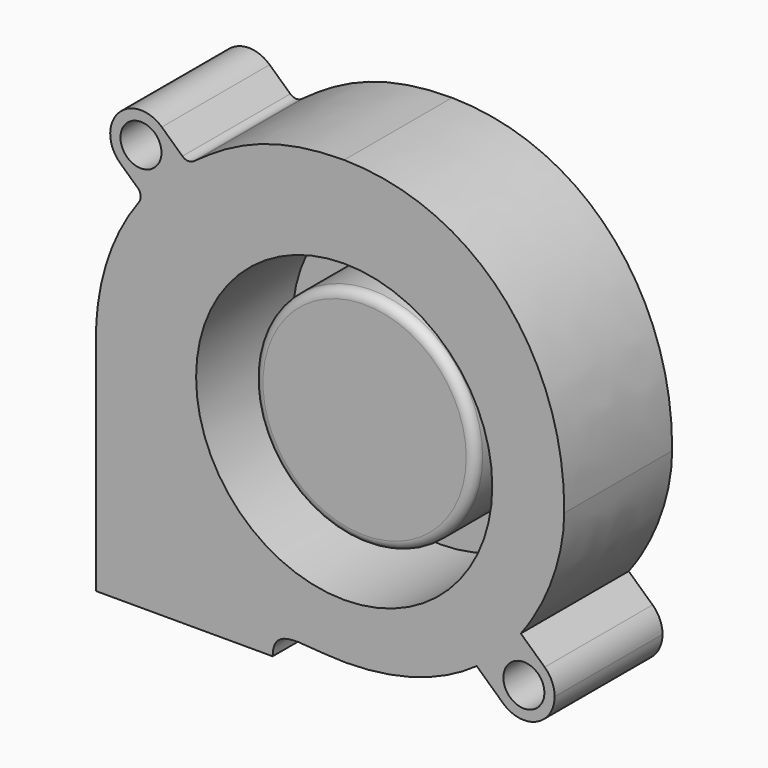
from build123d import *

# Parameters (mm, degrees)
F0_R     = 2.25
F1_DEPTH = 14.8
F0_R_2   = 12.15
F2_DEPTH = 1.6
F3_DEPTH = 12
F4_R     = 1
F5_W     = 17.4
F5_H     = 12.06
F6_DEPTH = 5


with BuildPart() as f1:
    # F0 (on Front) → F1 (new body)
    with BuildSketch(Plane.XZ):
        with BuildLine():
            Line((-27.25, 0), (-27.25, -24.25))
            Line((-27.25, -24.25), (-7.85, -24.25))
            add(Edge.make_bspline(
                [(-7.85, -24.25), (-7.8176427633, -20.8169110119), (-4.3375464156, -22.25), (0, -22.25)],
                knots=[0, 0, 0, 0, 8.1007715682, 8.1007715682, 8.1007715682, 8.1007715682], degree=3))
            add(Edge.make_bspline(
                [(14.5437740109, -17.909216005), (10.9068056005, -20.5097986935), (6.122203429, -22.25), (0, -22.25)],
                knots=[21.4185998801, 21.4185998801, 21.4185998801, 21.4185998801, 32.8372501894, 32.8372501894, 32.8372501894, 32.8372501894], degree=3))
            add(Edge.make_bspline(
                [(19.3821703567, -13.1875596661), (18.0720576154, -14.9154903789), (16.4686462302, -16.5328528348), (14.5437740109, -17.909216005)],
                knots=[15.3752582058, 15.3752582058, 15.3752582058, 15.3752582058, 21.4185998801, 21.4185998801, 21.4185998801, 21.4185998801], degree=3))
            add(Edge.make_bspline(
                [(24.15, 0), (24.15, -3.6795945823), (22.7153133033, -8.7914188713), (19.3821703567, -13.1875596661)],
                knots=[0, 0, 0, 0, 15.3752582058, 15.3752582058, 15.3752582058, 15.3752582058], degree=3))
            add(Edge.make_bspline(
                [(24.15, 0), (24.2929216474, 14.3250608817), (14.8955499753, 26.0717794299), (0, 26.25)],
                knots=[0, 0, 0, 0, 35.6691042781, 35.6691042781, 35.6691042781, 35.6691042781], degree=3))
            add(Edge.make_bspline(
                [(0, 26.25), (-5.135877891, 26.2629323961), (-11.114542158, 24.5071482084), (-16.161044046, 21.0100500089)],
                knots=[0, 0, 0, 0, 16.8847295513, 16.8847295513, 16.8847295513, 16.8847295513], degree=3))
            add(Edge.make_bspline(
                [(-16.161044046, 21.0100500089), (-16.2712231538, 20.9311478534), (-16.3801314978, 20.8526765927), (-16.487850408, 20.7747483814)],
                knots=[16.497992714, 16.497992714, 16.497992714, 16.497992714, 17.0339105302, 17.0339105302, 17.0339105302, 17.0339105302], degree=3))
            add(Edge.make_bspline(
                [(-16.487850408, 20.7747483814), (-16.7124834128, 20.6122397909), (-16.9319438817, 20.4520927797), (-17.1469693705, 20.2953244431)],
                knots=[17.0339105302, 17.0339105302, 17.0339105302, 17.0339105302, 18.1514935909, 18.1514935909, 18.1514935909, 18.1514935909], degree=3))
            add(Edge.make_bspline(
                [(-17.1469693705, 20.2953244431), (-19.1547308604, 18.7732329399), (-20.9874640515, 16.9609662016), (-22.5242380569, 14.8603912213)],
                knots=[17.9984458903, 17.9984458903, 17.9984458903, 17.9984458903, 24.8946681266, 24.8946681266, 24.8946681266, 24.8946681266], degree=3))
            add(Edge.make_bspline(
                [(-22.5242380569, 14.8603912213), (-25.4083045723, 10.9182384112), (-27.25, 5.9606612107), (-27.25, 0)],
                knots=[24.8946681266, 24.8946681266, 24.8946681266, 24.8946681266, 37.836820691, 37.836820691, 37.836820691, 37.836820691], degree=3))
        make_face()
        with BuildLine():
            ThreePointArc((16.25, 0), (-11.4904851943, -11.4904851943), (0, 16.25))
            ThreePointArc((0, 16.25), (11.4904851943, 11.4904851943), (16.25, 0))
        make_face(mode=Mode.SUBTRACT)
        with BuildLine():
            ThreePointArc((-22.6556099396, 16.1880189983), (-22.3361709954, 15.5493145647), (-22.5242380569, 14.8603912213))
            add(Edge.make_bspline(
                [(-17.1469693705, 20.2953244431), (-19.1547308604, 18.7732329399), (-20.9874640515, 16.9609662016), (-22.5242380569, 14.8603912213)],
                knots=[17.9984458903, 17.9984458903, 17.9984458903, 17.9984458903, 24.8946681266, 24.8946681266, 24.8946681266, 24.8946681266], degree=3))
            add(Edge.make_bspline(
                [(-16.5707430692, 20.7208158925), (-16.7643258601, 20.5815997135), (-16.9564357443, 20.4397686985), (-17.1469693705, 20.2953244431)],
                knots=[17.3440044956, 17.3440044956, 17.3440044956, 17.3440044956, 17.9984458903, 17.9984458903, 17.9984458903, 17.9984458903], degree=3))
            ThreePointArc((-16.5707430692, 20.7208158925), (-17.1810656026, 20.5907080667), (-17.7496903525, 20.8477830266))
            Line((-17.7496903525, 20.8477830266), (-20.0190790788, 22.927921795))
            ThreePointArc((-20.0190790788, 22.927921795), (-19.2102914227, 21.7989913577), (-18.924569733, 20.439953271))
            ThreePointArc((-18.924569733, 20.439953271), (-20.9405316464, 17.3506749607), (-24.5800603872, 17.9519847471))
            Line((-24.5800603872, 17.9519847471), (-22.6556099396, 16.1880189983))
        make_face()
        with BuildLine():
            add(Edge.make_bspline(
                [(19.3821703567, -13.1875596661), (18.0720576154, -14.9154903789), (16.4686462302, -16.5328528348), (14.5437740109, -17.909216005)],
                knots=[15.3752582058, 15.3752582058, 15.3752582058, 15.3752582058, 21.4185998801, 21.4185998801, 21.4185998801, 21.4185998801], degree=3))
            Line((14.5437740109, -17.909216005), (17.4389635725, -20.5629685239))
            ThreePointArc((17.4389635725, -20.5629685239), (17.2314857028, -15.7945093458), (21.9999448809, -15.5870314761))
            Line((21.9999448809, -15.5870314761), (19.3821703567, -13.1875596661))
        make_face()
        with BuildLine():
            add(Edge.make_bspline(
                [(-16.5707430692, 20.7208158925), (-16.7643258601, 20.5815997135), (-16.9564357443, 20.4397686985), (-17.1469693705, 20.2953244431)],
                knots=[17.3440044956, 17.3440044956, 17.3440044956, 17.3440044956, 17.9984458903, 17.9984458903, 17.9984458903, 17.9984458903], degree=3))
            add(Edge.make_bspline(
                [(-16.487850408, 20.7747483814), (-16.7124834128, 20.6122397909), (-16.9319438817, 20.4520927797), (-17.1469693705, 20.2953244431)],
                knots=[17.0339105302, 17.0339105302, 17.0339105302, 17.0339105302, 18.1514935909, 18.1514935909, 18.1514935909, 18.1514935909], degree=3))
            ThreePointArc((-16.487850408, 20.7747483814), (-16.5286296346, 20.7467568176), (-16.5707430692, 20.7208158925))
        make_face()
        with BuildLine():
            ThreePointArc((21.9999448809, -15.5870314761), (17.2314857028, -15.7945093458), (17.4389635725, -20.5629685239))
            ThreePointArc((17.4389635725, -20.5629685239), (21.0784923134, -21.1642783104), (23.0944542267, -18.075))
            ThreePointArc((23.0944542267, -18.075), (22.8087325371, -16.7159619133), (21.9999448809, -15.5870314761))
        make_face()
        with Locations((19.7194542267, -18.075)):
            Circle(F0_R, mode=Mode.SUBTRACT)
        with BuildLine():
            ThreePointArc((-20.0190790788, 22.927921795), (-24.787538257, 22.7204439252), (-24.5800603872, 17.9519847471))
            ThreePointArc((-24.5800603872, 17.9519847471), (-20.9405316464, 17.3506749607), (-18.924569733, 20.439953271))
            ThreePointArc((-18.924569733, 20.439953271), (-19.2102914227, 21.7989913577), (-20.0190790788, 22.927921795))
        make_face()
        with Locations((-22.299569733, 20.439953271)):
            Circle(F0_R, mode=Mode.SUBTRACT)
        with BuildLine():
            add(Edge.make_bspline(
                [(0, 26.25), (-8.1731251983, 26.2763401513), (-12.7692289915, 23.4390179358), (-16.161044046, 21.0100500089)],
                knots=[0, 0, 0, 0, 16.497992714, 16.497992714, 16.497992714, 16.497992714], degree=3))
            add(Edge.make_bspline(
                [(0, 26.25), (-5.135877891, 26.2629323961), (-11.114542158, 24.5071482084), (-16.161044046, 21.0100500089)],
                knots=[0, 0, 0, 0, 16.8847295513, 16.8847295513, 16.8847295513, 16.8847295513], degree=3))
        make_face()
    extrude(amount=F1_DEPTH)

    # F0 (on Front) → F2 (join)
    with BuildSketch(Plane.XZ):
        with BuildLine():
            Line((-27.25, 0), (-27.25, -24.25))
            Line((-27.25, -24.25), (-7.85, -24.25))
            add(Edge.make_bspline(
                [(-7.85, -24.25), (-7.8176427633, -20.8169110119), (-4.3375464156, -22.25), (0, -22.25)],
                knots=[0, 0, 0, 0, 8.1007715682, 8.1007715682, 8.1007715682, 8.1007715682], degree=3))
            add(Edge.make_bspline(
                [(14.5437740109, -17.909216005), (10.9068056005, -20.5097986935), (6.122203429, -22.25), (0, -22.25)],
                knots=[21.4185998801, 21.4185998801, 21.4185998801, 21.4185998801, 32.8372501894, 32.8372501894, 32.8372501894, 32.8372501894], degree=3))
            add(Edge.make_bspline(
                [(19.3821703567, -13.1875596661), (18.0720576154, -14.9154903789), (16.4686462302, -16.5328528348), (14.5437740109, -17.909216005)],
                knots=[15.3752582058, 15.3752582058, 15.3752582058, 15.3752582058, 21.4185998801, 21.4185998801, 21.4185998801, 21.4185998801], degree=3))
            add(Edge.make_bspline(
                [(24.15, 0), (24.15, -3.6795945823), (22.7153133033, -8.7914188713), (19.3821703567, -13.1875596661)],
                knots=[0, 0, 0, 0, 15.3752582058, 15.3752582058, 15.3752582058, 15.3752582058], degree=3))
            add(Edge.make_bspline(
                [(24.15, 0), (24.2929216474, 14.3250608817), (14.8955499753, 26.0717794299), (0, 26.25)],
                knots=[0, 0, 0, 0, 35.6691042781, 35.6691042781, 35.6691042781, 35.6691042781], degree=3))
            add(Edge.make_bspline(
                [(0, 26.25), (-5.135877891, 26.2629323961), (-11.114542158, 24.5071482084), (-16.161044046, 21.0100500089)],
                knots=[0, 0, 0, 0, 16.8847295513, 16.8847295513, 16.8847295513, 16.8847295513], degree=3))
            add(Edge.make_bspline(
                [(-16.161044046, 21.0100500089), (-16.2712231538, 20.9311478534), (-16.3801314978, 20.8526765927), (-16.487850408, 20.7747483814)],
                knots=[16.497992714, 16.497992714, 16.497992714, 16.497992714, 17.0339105302, 17.0339105302, 17.0339105302, 17.0339105302], degree=3))
            add(Edge.make_bspline(
                [(-16.487850408, 20.7747483814), (-16.7124834128, 20.6122397909), (-16.9319438817, 20.4520927797), (-17.1469693705, 20.2953244431)],
                knots=[17.0339105302, 17.0339105302, 17.0339105302, 17.0339105302, 18.1514935909, 18.1514935909, 18.1514935909, 18.1514935909], degree=3))
            add(Edge.make_bspline(
                [(-17.1469693705, 20.2953244431), (-19.1547308604, 18.7732329399), (-20.9874640515, 16.9609662016), (-22.5242380569, 14.8603912213)],
                knots=[17.9984458903, 17.9984458903, 17.9984458903, 17.9984458903, 24.8946681266, 24.8946681266, 24.8946681266, 24.8946681266], degree=3))
            add(Edge.make_bspline(
                [(-22.5242380569, 14.8603912213), (-25.4083045723, 10.9182384112), (-27.25, 5.9606612107), (-27.25, 0)],
                knots=[24.8946681266, 24.8946681266, 24.8946681266, 24.8946681266, 37.836820691, 37.836820691, 37.836820691, 37.836820691], degree=3))
        make_face()
        with BuildLine():
            ThreePointArc((16.25, 0), (-11.4904851943, -11.4904851943), (0, 16.25))
            ThreePointArc((0, 16.25), (11.4904851943, 11.4904851943), (16.25, 0))
        make_face(mode=Mode.SUBTRACT)
        with BuildLine():
            ThreePointArc((16.25, 0), (11.4904851943, 11.4904851943), (0, 16.25))
            ThreePointArc((0, 16.25), (-11.4904851943, -11.4904851943), (16.25, 0))
        make_face()
        Circle(F0_R_2, mode=Mode.SUBTRACT)
        Circle(F0_R_2)
        with BuildLine():
            ThreePointArc((-20.0190790788, 22.927921795), (-24.787538257, 22.7204439252), (-24.5800603872, 17.9519847471))
            ThreePointArc((-24.5800603872, 17.9519847471), (-20.9405316464, 17.3506749607), (-18.924569733, 20.439953271))
            ThreePointArc((-18.924569733, 20.439953271), (-19.2102914227, 21.7989913577), (-20.0190790788, 22.927921795))
        make_face()
        with Locations((-22.299569733, 20.439953271)):
            Circle(F0_R, mode=Mode.SUBTRACT)
        with BuildLine():
            ThreePointArc((21.9999448809, -15.5870314761), (17.2314857028, -15.7945093458), (17.4389635725, -20.5629685239))
            ThreePointArc((17.4389635725, -20.5629685239), (21.0784923134, -21.1642783104), (23.0944542267, -18.075))
            ThreePointArc((23.0944542267, -18.075), (22.8087325371, -16.7159619133), (21.9999448809, -15.5870314761))
        make_face()
        with Locations((19.7194542267, -18.075)):
            Circle(F0_R, mode=Mode.SUBTRACT)
        with BuildLine():
            add(Edge.make_bspline(
                [(19.3821703567, -13.1875596661), (18.0720576154, -14.9154903789), (16.4686462302, -16.5328528348), (14.5437740109, -17.909216005)],
                knots=[15.3752582058, 15.3752582058, 15.3752582058, 15.3752582058, 21.4185998801, 21.4185998801, 21.4185998801, 21.4185998801], degree=3))
            Line((14.5437740109, -17.909216005), (17.4389635725, -20.5629685239))
            ThreePointArc((17.4389635725, -20.5629685239), (17.2314857028, -15.7945093458), (21.9999448809, -15.5870314761))
            Line((21.9999448809, -15.5870314761), (19.3821703567, -13.1875596661))
        make_face()
    extrude(amount=F2_DEPTH)

    # F0 (on Front) → F3 (join)
    with BuildSketch(Plane.XZ):
        Circle(F0_R_2)
    extrude(amount=F3_DEPTH)

    # F4
    f4_edges = [f1.edges().sort_by_distance(p)[0] for p in [
        (-12.15, -12, 0),
    ]]
    fillet(f4_edges, radius=F4_R)

    # F5 (on face) → F6 (cut)
    with BuildSketch(Plane(origin=(0, 0, -24.25), x_dir=(1, 0, 0), z_dir=(0, 0, -1))):
        with Locations((-17.55, 7.63)):
            Rectangle(F5_W, F5_H)
    extrude(amount=-F6_DEPTH, mode=Mode.SUBTRACT)


solid = f1.part
